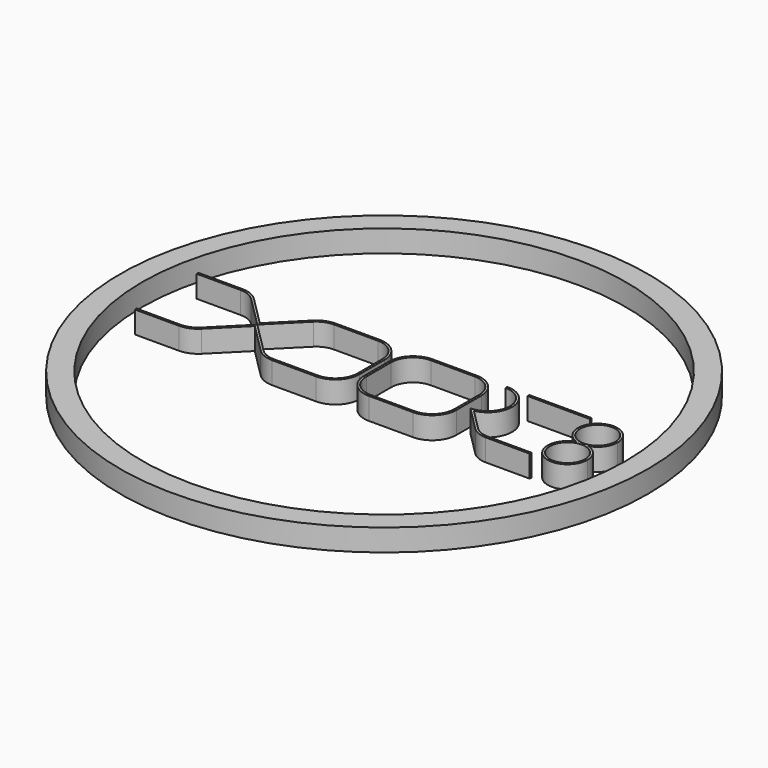
from build123d import *

# Parameters (mm, degrees)
F0_W     = 0.5
F0_H     = 7.0710678119
F1_DEPTH = 5
F0_W_2   = 14.1421356237
F0_H_2   = 0.5
F0_R     = 4
F0_R_2   = 60
F0_R_3   = 55


# Not quite as in the source:
# - a feature names something its author has since deleted; it is built from what else it names


with BuildPart() as f1:
    # F0 (on Top) → F1 (new body)
    with BuildSketch(Plane.XY):
        with BuildLine():
            ThreePointArc((-10.6066017178, 8.5355339059), (-8.693184556, 8.1549315685), (-7.0710678119, 7.0710678119))
            Line((-7.0710678119, 7.0710678119), (-0.01, 0.01))
            Line((-0.01, 0.01), (0, 0))
            Line((0, 0), (0, 0.7071067812))
            Line((0, 0.7071067812), (-6.7175144213, 7.4246212025))
            ThreePointArc((-6.7175144213, 7.4246212025), (-8.5018428398, 8.6168713347), (-10.6066017178, 9.0355339059))
            Line((-10.6066017178, 9.0355339059), (-20.6066017178, 9.0355339059))
            Line((-20.6066017178, 9.0355339059), (-20.6066017178, 8.5355339059))
            Line((-20.6066017178, 8.5355339059), (-10.6066017178, 8.5355339059))
        make_face()
        Polygon((0, 0), (-0.01, 0.01), (-0.01, -0.01), align=None)
        with BuildLine():
            Line((0, -0.7071067812), (0, 0))
            Line((0, 0), (-0.01, -0.01))
            Line((-0.01, -0.01), (-7.0710678119, -7.0710678119))
            ThreePointArc((-7.0710678119, -7.0710678119), (-8.693184556, -8.1549315685), (-10.6066017178, -8.5355339059))
            Line((-10.6066017178, -8.5355339059), (-20.6066017178, -8.5355339059))
            Line((-20.6066017178, -8.5355339059), (-20.6066017178, -9.0355339059))
            Line((-20.6066017178, -9.0355339059), (-10.6066017178, -9.0355339059))
            ThreePointArc((-10.6066017178, -9.0355339059), (-8.5018428398, -8.6168713347), (-6.7175144213, -7.4246212025))
            Line((-6.7175144213, -7.4246212025), (0, -0.7071067812))
        make_face()
        with BuildLine():
            Line((0, 0.7071067812), (0, 0))
            Line((0, 0), (0.01, 0.01))
            Line((0.01, 0.01), (7.0710678119, 7.0710678119))
            ThreePointArc((7.0710678119, 7.0710678119), (8.693184556, 8.1549315685), (10.6066017178, 8.5355339059))
            Line((10.6066017178, 8.5355339059), (20.6066017178, 8.5355339059))
            ThreePointArc((20.6066017178, 8.5355339059), (24.1421356237, 7.0710678119), (25.6066017178, 3.5355339059))
            Line((25.6066017178, 3.5355339059), (26.1066017178, 3.5355339059))
            ThreePointArc((26.1066017178, 3.5355339059), (24.4956890143, 7.4246212025), (20.6066017178, 9.0355339059))
            Line((20.6066017178, 9.0355339059), (10.6066017178, 9.0355339059))
            ThreePointArc((10.6066017178, 9.0355339059), (8.5018428398, 8.6168713347), (6.7175144213, 7.4246212025))
            Line((6.7175144213, 7.4246212025), (0, 0.7071067812))
        make_face()
        Polygon((0.01, 0.01), (0, 0), (0.01, -0.01), align=None)
        with BuildLine():
            Line((0.01, -0.01), (0, 0))
            Line((0, 0), (0, -0.7071067812))
            Line((0, -0.7071067812), (6.7175144213, -7.4246212025))
            ThreePointArc((6.7175144213, -7.4246212025), (8.5018428398, -8.6168713347), (10.6066017178, -9.0355339059))
            Line((10.6066017178, -9.0355339059), (20.6066017178, -9.0355339059))
            ThreePointArc((20.6066017178, -9.0355339059), (24.4956890143, -7.4246212025), (26.1066017178, -3.5355339059))
            Line((26.1066017178, -3.5355339059), (25.6066017178, -3.5355339059))
            ThreePointArc((25.6066017178, -3.5355339059), (24.1421356237, -7.0710678119), (20.6066017178, -8.5355339059))
            Line((20.6066017178, -8.5355339059), (10.6066017178, -8.5355339059))
            ThreePointArc((10.6066017178, -8.5355339059), (8.693184556, -8.1549315685), (7.0710678119, -7.0710678119))
            Line((7.0710678119, -7.0710678119), (0.01, -0.01))
        make_face()
        with Locations((25.8566017178, 0)):
            Rectangle(F0_W, F0_H)
    extrude(amount=F1_DEPTH)


with BuildPart() as f1b:
    # F0 (on Top) → F1, piece 2 (new body)
    with BuildSketch(Plane.XY):
        with BuildLine():
            ThreePointArc((49.6066017178, 8.5355339059), (54.6066017178, 3.5355339059), (49.6066017178, -1.4644660941))
            Line((49.6066017178, -1.4644660941), (55.2132034356, -7.0710678119))
            ThreePointArc((55.2132034356, -7.0710678119), (56.8353201797, -8.1549315685), (58.7487373415, -8.5355339059))
            Line((58.7487373415, -8.5355339059), (68.7487373415, -8.5355339059))
            Line((68.7487373415, -8.5355339059), (68.7487373415, -8.0355339059))
            Line((68.7487373415, -8.0355339059), (58.7487373415, -8.0355339059))
            ThreePointArc((58.7487373415, -8.0355339059), (57.0266618959, -7.6929918022), (55.5667568262, -6.7175144213))
            Line((55.5667568262, -6.7175144213), (50.7032657992, -1.8540233943))
            ThreePointArc((50.7032657992, -1.8540233943), (55.0789213883, 4.086639544), (49.6066017178, 9.0355339059))
            Line((49.6066017178, 9.0355339059), (49.6066017178, 8.5355339059))
        make_face()
    extrude(amount=F1_DEPTH)


with BuildPart() as f1c:
    # F0 (on Top) → F1, piece 3 (new body)
    with BuildSketch(Plane.XY):
        with Locations((61.6776695297, 8.7855339059)):
            Rectangle(F0_W_2, F0_H_2)
    extrude(amount=F1_DEPTH)


with BuildPart() as f1d:
    # F0 (on Top) → F1, piece 4 (new body)
    with BuildSketch(Plane.XY):
        with BuildLine():
            ThreePointArc((72.3760760063, 0.25), (71.0960948862, -7.6705700824), (78.2487373415, -4.0355339059))
            ThreePointArc((78.2487373415, -4.0355339059), (77.383773518, -1.3828914506), (75.1213986767, 0.25))
            ThreePointArc((75.1213986767, 0.25), (73.7487373415, 0.0355339059), (72.3760760063, 0.25))
        make_face()
        with Locations((73.7487373415, -4.0355339059)):
            Circle(F0_R, mode=Mode.SUBTRACT)
        with BuildLine():
            ThreePointArc((72.3760760063, 0.25), (73.7487373415, 0.0355339059), (75.1213986767, 0.25))
            ThreePointArc((75.1213986767, 0.25), (73.7487373415, 0.4644660941), (72.3760760063, 0.25))
        make_face()
        with BuildLine():
            ThreePointArc((72.3760760063, 0.25), (73.7487373415, 0.4644660941), (75.1213986767, 0.25))
            ThreePointArc((75.1213986767, 0.25), (77.383773518, 1.8828914506), (78.2487373415, 4.5355339059))
            ThreePointArc((78.2487373415, 4.5355339059), (71.0960948862, 8.1705700824), (72.3760760063, 0.25))
        make_face()
        with Locations((73.7487373415, 4.5355339059)):
            Circle(F0_R, mode=Mode.SUBTRACT)
    extrude(amount=F1_DEPTH)


with BuildPart() as f1e:
    # F0 (on Top) → F1, piece 5 (new body)
    with BuildSketch(Plane.XY):
        with BuildLine():
            Line((42.6066017178, 9.0355339059), (32.6066017178, 9.0355339059))
            ThreePointArc((32.6066017178, 9.0355339059), (28.7175144213, 7.4246212025), (27.1066017178, 3.5355339059))
            Line((27.1066017178, 3.5355339059), (27.1066017178, -3.5355339059))
            ThreePointArc((27.1066017178, -3.5355339059), (28.7175144213, -7.4246212025), (32.6066017178, -9.0355339059))
            Line((32.6066017178, -9.0355339059), (42.6066017178, -9.0355339059))
            ThreePointArc((42.6066017178, -9.0355339059), (46.4956890143, -7.4246212025), (48.1066017178, -3.5355339059))
            Line((48.1066017178, -3.5355339059), (48.1066017178, 3.5355339059))
            ThreePointArc((48.1066017178, 3.5355339059), (46.4956890143, 7.4246212025), (42.6066017178, 9.0355339059))
        make_face()
        with BuildLine():
            Line((27.6066017178, -3.5355339059), (27.6066017178, 3.5355339059))
            ThreePointArc((27.6066017178, 3.5355339059), (29.0710678119, 7.0710678119), (32.6066017178, 8.5355339059))
            Line((32.6066017178, 8.5355339059), (42.6066017178, 8.5355339059))
            ThreePointArc((42.6066017178, 8.5355339059), (46.1421356237, 7.0710678119), (47.6066017178, 3.5355339059))
            Line((47.6066017178, 3.5355339059), (47.6066017178, -3.5355339059))
            ThreePointArc((47.6066017178, -3.5355339059), (46.1421356237, -7.0710678119), (42.6066017178, -8.5355339059))
            Line((42.6066017178, -8.5355339059), (32.6066017178, -8.5355339059))
            ThreePointArc((32.6066017178, -8.5355339059), (29.0710678119, -7.0710678119), (27.6066017178, -3.5355339059))
        make_face(mode=Mode.SUBTRACT)
    extrude(amount=F1_DEPTH)


with BuildPart() as f1f:
    # F0 (on Top) → F1, piece 6 (new body)
    with BuildSketch(Plane.XY):
        with Locations((28.8208982822, -3.39059e-05)):
            Circle(F0_R_2)
        with Locations((28.8208982822, -3.39059e-05)):
            Circle(F0_R_3, mode=Mode.SUBTRACT)
    extrude(amount=F1_DEPTH)


solid = Compound([f1.part, f1b.part, f1c.part, f1d.part, f1e.part, f1f.part])
